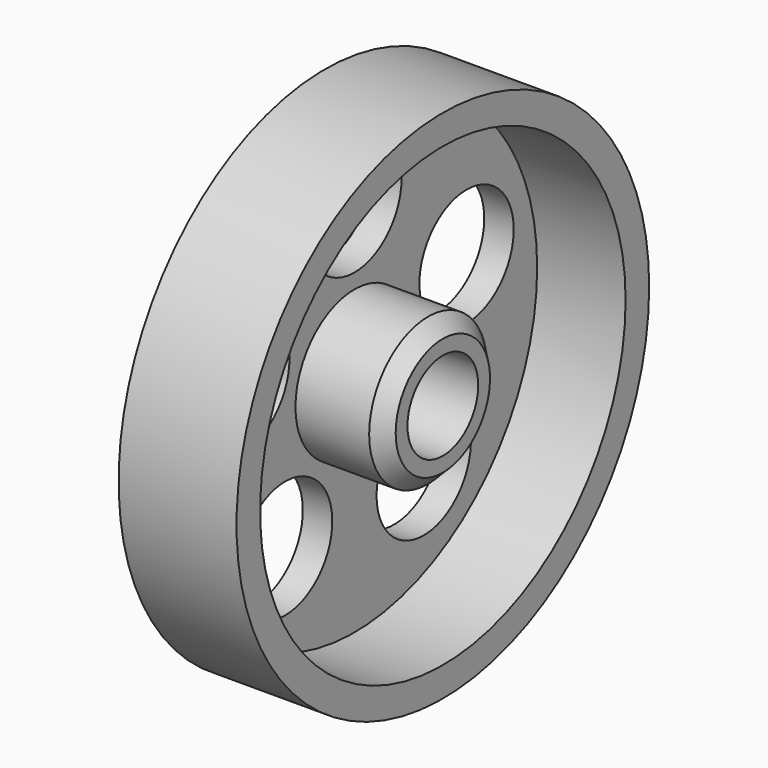
from build123d import *

# Parameters (mm, degrees)
F0_W            = 8
F0_H            = 17.5
F3_D            = 6
F4_T            = -2
F6_D            = 8
F6_COPIES_COUNT = 5
F7_SIZE         = 1


# Not quite as in the source:
# - a pattern or mirror of a feature is missing from the dataset's text; its kind, count and spacing are read off the source's solid


with BuildPart() as f1:
    # F0 (on Top) → F1 (revolve)
    with BuildSketch(Plane.XY):
        with Locations((4, 8.75)):
            Rectangle(F0_W, F0_H)
    revolve(axis=Axis((4, 0, 0), (1, 0, 0)))

    # F3 (through all)
    with Locations(Plane(origin=(0, 0, 0), x_dir=(0, 1, 0), z_dir=(-1, 0, 0))):
        with Locations((0, 0)):
            Hole(F3_D / 2)

    # F4
    f4_openings = [f1.faces().sort_by_distance(p)[0] for p in [
        (8, -17.005025, 0),
    ]]
    offset(amount=F4_T, openings=f4_openings)

    # F6 (through all)
    with Locations(Plane(origin=(0, 0, 0), x_dir=(0, -1, 0), z_dir=(-1, 0, 0))):
        with Locations((0, 10)):
            f6 = Hole(F6_D / 2)

    # F6_copies: F6 ×5 about axis
    f6_copies_axis = Axis((0, 0, 0), (1, 0, 0))
    for i in range(1, F6_COPIES_COUNT):
        add(f6.rotate(f6_copies_axis, i * 360 / F6_COPIES_COUNT), mode=Mode.SUBTRACT)

    # F7
    f7_edges = [f1.edges().sort_by_distance(p)[0] for p in [
        (8, -5, 0),
    ]]
    chamfer(f7_edges, length=F7_SIZE)


solid = f1.part
